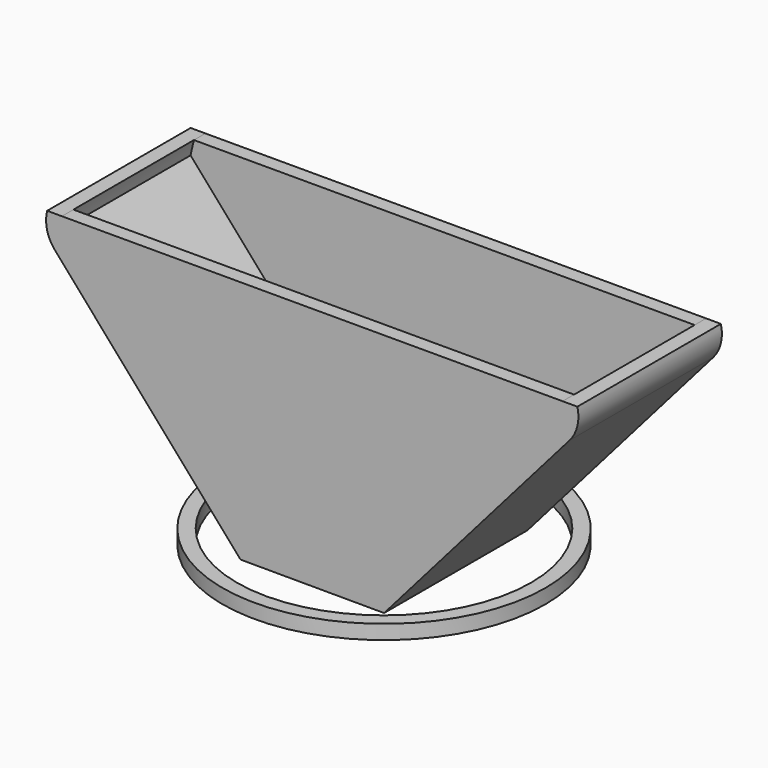
from build123d import *

# Parameters (mm, degrees)
F0_R     = 22.5
F0_R_2   = 20.5
F1_DEPTH = 2
F3_DEPTH = 12.5
F4_DEPTH = 10.5


with BuildPart() as f1:
    # F0 (on Top) → F1 (new body)
    with BuildSketch(Plane.XY):
        Circle(F0_R)
        Circle(F0_R_2, mode=Mode.SUBTRACT)
    extrude(amount=F1_DEPTH)


with BuildPart() as f3:
    # F2 (on Front) → F3 (new body, symmetric)
    with BuildSketch(Plane.XZ):
        with BuildLine():
            ThreePointArc((35.8647954681, 29.5480771848), (36.9575138291, 31.6563697), (36.9543489902, 34.0310108793))
            Line((36.9543489902, 34.0310108793), (35.3566579925, 32.0066029077))
            Line((35.3566579925, 32.0066029077), (7.3626854021, -0.0445880533))
            Line((7.3626854021, -0.0445880533), (10.0121919702, -0.0513920895))
            Line((10.0121919702, -0.0513920895), (35.8647954681, 29.5480771848))
        make_face()
        with BuildLine():
            Line((35.3566579925, 32.0066029077), (36.9543489902, 34.0310108793))
            Line((36.9543489902, 34.0310108793), (34.8912937434, 34.031108467))
            ThreePointArc((34.8912937434, 34.031108467), (35.1385591119, 33.022207874), (35.3566579925, 32.0066029077))
        make_face()
        with BuildLine():
            Line((7.3626854021, -0.0445880533), (35.3566579925, 32.0066029077))
            ThreePointArc((35.3566579925, 32.0066029077), (35.1385591119, 33.022207874), (34.8912937434, 34.031108467))
            Line((34.8912937434, 34.031108467), (-34.8904340011, 34.0344093193))
            ThreePointArc((-34.8904340011, 34.0344093193), (-35.1380360371, 33.0244831042), (-35.3564115486, 32.0078367231))
            Line((-35.3564115486, 32.0078367231), (-7.3361719456, -0.0068408143))
            Line((-7.3361719456, -0.0068408143), (7.3626854021, -0.0445880533))
        make_face()
        with BuildLine():
            Line((-35.3564115486, 32.0078367231), (-36.953489248, 34.0345069071))
            ThreePointArc((-36.953489248, 34.0345069071), (-36.9562144908, 31.6571352246), (-35.8606602894, 29.5472384177))
            Line((-35.8606602894, 29.5472384177), (-10, 0))
            Line((-10, 0), (-7.3361719456, -0.0068408143))
            Line((-7.3361719456, -0.0068408143), (-35.3564115486, 32.0078367231))
        make_face()
        with BuildLine():
            Line((-34.8904340011, 34.0344093193), (-36.953489248, 34.0345069071))
            Line((-36.953489248, 34.0345069071), (-35.3564115486, 32.0078367231))
            ThreePointArc((-35.3564115486, 32.0078367231), (-35.1380360371, 33.0244831042), (-34.8904340011, 34.0344093193))
        make_face()
    extrude(amount=F3_DEPTH, both=True)

    # F2 (on Front) → F4 (cut, symmetric)
    with BuildSketch(Plane.XZ):
        with BuildLine():
            ThreePointArc((8.42e-08, 63), (23.4777886852, 54.8945488781), (36.9543489902, 34.0310108793))
            Line((36.9543489902, 34.0310108793), (36.9557192967, 63))
            Line((36.9557192967, 63), (8.42e-08, 63))
        make_face()
        with BuildLine():
            Line((7.3626854021, -0.0445880533), (35.3566579925, 32.0066029077))
            ThreePointArc((35.3566579925, 32.0066029077), (35.1385591119, 33.022207874), (34.8912937434, 34.031108467))
            Line((34.8912937434, 34.031108467), (-34.8904340011, 34.0344093193))
            ThreePointArc((-34.8904340011, 34.0344093193), (-35.1380360371, 33.0244831042), (-35.3564115486, 32.0078367231))
            Line((-35.3564115486, 32.0078367231), (-7.3361719456, -0.0068408143))
            Line((-7.3361719456, -0.0068408143), (7.3626854021, -0.0445880533))
        make_face()
    extrude(amount=F4_DEPTH, both=True, mode=Mode.SUBTRACT)


solid = Compound([f1.part, f3.part])
